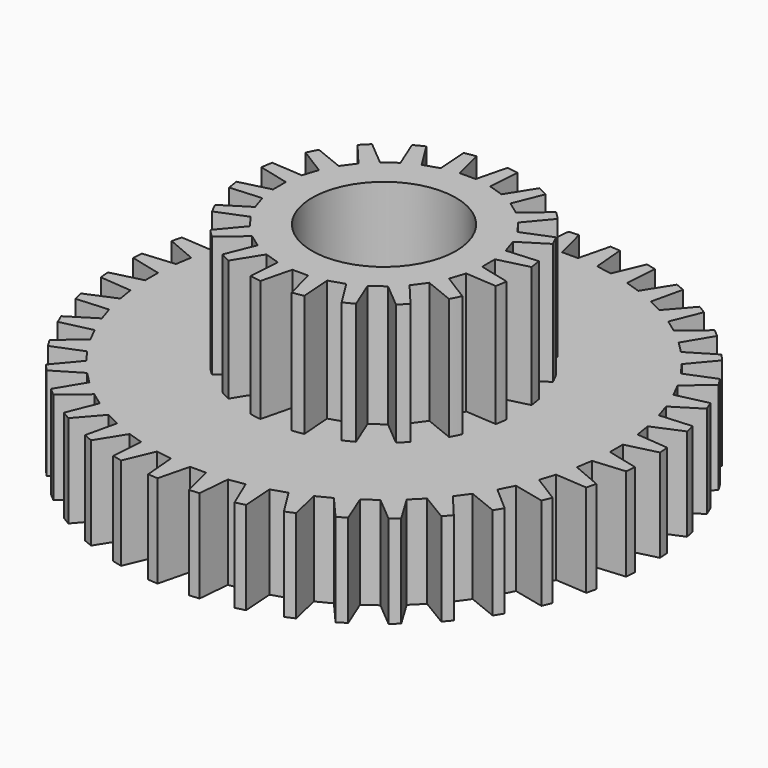
from build123d import *

# Parameters (mm, degrees)
F0_R            = 8.25
F1_DEPTH        = 2.9
F2_R            = 4.25
F3_DEPTH        = 3.8
F5_DEPTH        = 2.9
F5_COPIES_COUNT = 40
F8_DEPTH        = 3.8
F9_COUNT        = 20
F9_ANGLE        = 342
F10_R           = 2.25
F11_DEPTH       = 6.7
F10_R_2         = 6.9020481578
F10_R_3         = 4.9020481578
F10_R_4         = 3.9020481578
F10_R_5         = 2.9020481578
F12_DEPTH       = 0.5


# Not quite as in the source:
# - a feature of the source that left no trace in its solid (it failed there, or was rolled back) is left out
# - a pattern or mirror of a feature is missing from the dataset's text; its kind, count and spacing are read off the source's solid


with BuildPart() as f1:
    # F0 (on Top) → F1 (new body)
    with BuildSketch(Plane.XY):
        Circle(F0_R)
    extrude(amount=F1_DEPTH)

    # F2 (on face) → F3 (join)
    with BuildSketch(Plane.XY.offset(2.9)):
        Circle(F2_R)
    extrude(amount=F3_DEPTH)

    # F4 (on face) → F5 (cut)
    with BuildSketch(Plane.XY.offset(2.9)):
        with BuildLine():
            ThreePointArc((0.4919195185, 8.2353211952), (0, 8.25), (-0.4919195185, 8.2353211952))
            Line((-0.4919195185, 8.2353211952), (-0.25, 7.265035003))
            Line((-0.25, 7.265035003), (0.25, 7.265035003))
            Line((0.25, 7.265035003), (0.4919195185, 8.2353211952))
        make_face()
    f5 = extrude(amount=-F5_DEPTH, mode=Mode.SUBTRACT)

    # F5_copies: F5 ×40 about axis
    f5_copies_axis = Axis((0, 0, 0), (0, 0, 1))
    for i in range(1, F5_COPIES_COUNT):
        add(f5.rotate(f5_copies_axis, i * 360 / F5_COPIES_COUNT), mode=Mode.SUBTRACT)

    # F7 (on face) → F8 (cut)
    with BuildSketch(Plane.XY.offset(6.7)):
        with BuildLine():
            ThreePointArc((0.4875978882, 4.221936558), (0, 4.25), (-0.4875978882, 4.221936558))
            Line((-0.4875978882, 4.221936558), (-0.25, 3.2689834782))
            Line((-0.25, 3.2689834782), (0.25, 3.2689834782))
            Line((0.25, 3.2689834782), (0.4875978882, 4.221936558))
        make_face()
    f8 = extrude(amount=-F8_DEPTH, mode=Mode.SUBTRACT)

    # F9: F8 ×20 about axis
    f9_axis = Axis((0, 0, 2.9), (0, 0, -1))
    for i in range(1, F9_COUNT):
        add(f8.rotate(f9_axis, i * F9_ANGLE / (F9_COUNT - 1)), mode=Mode.SUBTRACT)

    # F10 (on face) → F11 (cut)
    with BuildSketch(Plane(origin=(0, 0, 0), x_dir=(1, 0, 0), z_dir=(0, 0, -1))):
        Circle(F10_R)
    extrude(amount=-F11_DEPTH, mode=Mode.SUBTRACT)

    # F10 (on face) → F12 (cut)
    with BuildSketch(Plane(origin=(0, 0, 0), x_dir=(1, 0, 0), z_dir=(0, 0, -1))):
        Circle(F10_R_2)
        Circle(F10_R_3, mode=Mode.SUBTRACT)
        Circle(F10_R_4)
        Circle(F10_R_5, mode=Mode.SUBTRACT)
    extrude(amount=-F12_DEPTH, mode=Mode.SUBTRACT)


solid = f1.part
